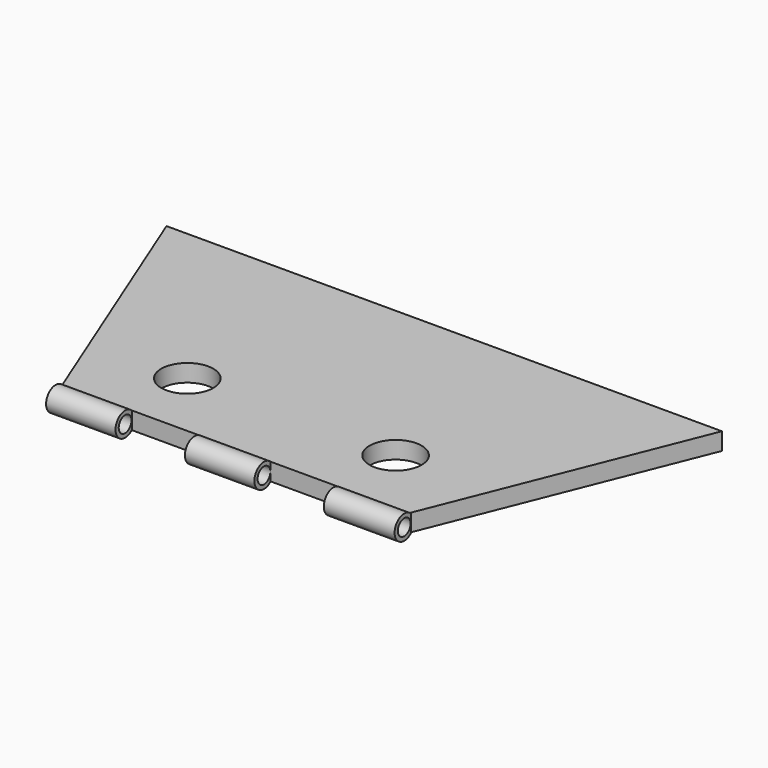
from build123d import *

# Parameters (mm, degrees)
F1_DEPTH      = 6.35
F2_R          = 2.921
F3_DEPTH      = 102.108
F3_DEPTH_BACK = 25.4
F6_D          = 19.05
F7_W          = 25.4
F7_H          = 8.6004827172
F7_H_2        = 11.8143679574
F8_DEPTH      = 12.7


# Not quite as in the source:
# - a feature names something its author has since deleted; it is built from what else it names


with BuildPart() as f1:
    # F0 (on Top) → F1 (new body)
    with BuildSketch(Plane.XY):
        Polygon((139.7, 95.25), (-63.5, 95.25), (-25.4, 0), (101.6, 0), align=None)
    extrude(amount=F1_DEPTH)

    # F2 (on Right) → F3 (join, two sides)
    with BuildSketch(Plane.YZ) as f3_sk:
        with BuildLine():
            Line((0, 0), (0, 6.337816827))
            ThreePointArc((0, 6.337816827), (-7.4383769178, 3.1689084135), (0, 0))
        make_face()
        with Locations((-3.0441769178, 3.1689084135)):
            Circle(F2_R, mode=Mode.SUBTRACT)
    extrude(amount=F3_DEPTH)
    extrude(f3_sk.sketch, amount=-F3_DEPTH_BACK)

    # F6 (through all)
    with Locations(Plane(origin=(0, 0, 0), x_dir=(1, 0, 0), z_dir=(0, 0, -1))):
        with Locations((0, -25.400012026), (76.2, -25.400012026)):
            Hole(F6_D / 2)

    # F7 (on face) → F8 (cut, symmetric)
    with BuildSketch(Plane.XY.offset(6.35)):
        with Locations((12.7, -4.3002413586)):
            Rectangle(F7_W, F7_H)
        with Locations((63.5, -5.9071839787)):
            Rectangle(F7_W, F7_H_2)
    extrude(amount=F8_DEPTH, both=True, mode=Mode.SUBTRACT)


solid = f1.part
